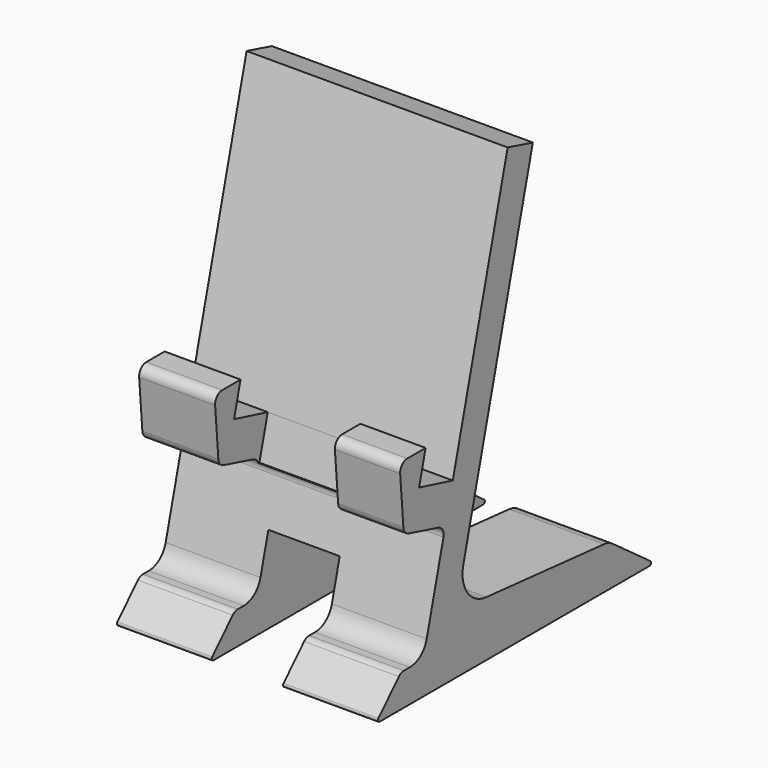
from build123d import *

# Parameters (mm, degrees)
F0_W     = 76.2
F0_H     = 101.6
F1_DEPTH = 133.35
F3_DEPTH = 76.201
F4_W     = 34.9662494294
F4_H     = 12.1309220302
F5_DEPTH = 25.4
F6_W     = 20.8403859288
F6_H     = 113.2664903998
F7_DEPTH = 25.4


# Not quite as in the source:
# - a feature names something its author has since deleted; it is built from what else it names


with BuildPart() as f1:
    # F0 (on Top) → F1 (new body)
    with BuildSketch(Plane.XY):
        Rectangle(F0_W, F0_H)
    extrude(amount=F1_DEPTH)

    # F2 (on face) → F3 (cut, through all)
    with BuildSketch(Plane.YZ.offset(38.1)):
        with BuildLine():
            Line((49.114014449, 0), (50.8, 0))
            Line((50.8, 0), (50.8, 66.2650913))
            Line((50.8, 66.2650913), (50.8, 73.7310647964))
            Line((50.8, 73.7310647964), (50.8, 128.6014442141))
            Line((50.8, 128.6014442141), (50.8, 133.35))
            Line((50.8, 133.35), (-50.8, 133.35))
            Line((-50.8, 133.35), (-50.8, 0))
            Line((-50.8, 0), (-49.3153884285, 0))
            ThreePointArc((-49.3153884285, 0), (-49.8930613229, 0.38308634), (-49.7649416709, 1.0642959051))
            Line((-49.7649416709, 1.0642959051), (-42.2846688887, 8.7558660005))
            ThreePointArc((-42.2846688887, 8.7558660005), (-41.4521127702, 9.3248290153), (-40.4637807514, 9.525))
            Line((-40.4637807514, 9.525), (-38.2985454719, 9.525))
            ThreePointArc((-38.2985454719, 9.525), (-34.4105014329, 10.8544807489), (-32.1505139925, 14.2862240786))
            Line((-32.1505139925, 14.2862240786), (-26.0325690106, 37.9606251271))
            ThreePointArc((-26.0325690106, 37.9606251271), (-26.3063034957, 39.9399780989), (-27.8936985581, 41.1536278306))
            Line((-27.8936985581, 41.1536278306), (-38.7149990474, 44.0606170611))
            ThreePointArc((-38.7149990474, 44.0606170611), (-40.050293777, 44.9146793042), (-40.6508289049, 46.3815780362))
            Line((-40.6508289049, 46.3815780362), (-41.828178264, 60.7104246977))
            ThreePointArc((-41.828178264, 60.7104246977), (-41.1424179273, 62.7046091009), (-39.2110885015, 63.5513707689))
            Line((-39.2110885015, 63.5513707689), (-32.5366084985, 63.5513707689))
            Line((-32.5366084985, 63.5513707689), (-34.9197723805, 54.3293235498))
            Line((-34.9197723805, 54.3293235498), (-22.6237094217, 51.1517717071))
            Line((-22.6237094217, 51.1517717071), (-2.6091445634, 128.6014442141))
            Line((-2.6091445634, 128.6014442141), (6.5897179326, 126.1302999894))
            Line((6.5897179326, 126.1302999894), (-18.753958765, 28.0587468857))
            ThreePointArc((-18.753958765, 28.0587468857), (-17.3156963729, 20.1857452314), (-10.3820422123, 16.1885970308))
            Line((-10.3820422123, 16.1885970308), (32.5785662344, 12.338888515))
            ThreePointArc((32.5785662344, 12.338888515), (34.2472884437, 11.9577274025), (35.7535762689, 11.144699363))
            Line((35.7535762689, 11.144699363), (49.5238091926, 1.1017641769))
            ThreePointArc((49.5238091926, 1.1017641769), (49.7017678057, 0.4084810434), (49.114014449, 0))
        make_face()
    extrude(amount=-F3_DEPTH, mode=Mode.SUBTRACT)

    # F4 (on face) → F5 (cut)
    with BuildSketch(Plane(origin=(0, -33.598613666, 8.682562632), x_dir=(1, 0, 0), z_dir=(0, -0.9681939338, 0.2502009325))):
        Polygon((19.05, 73.9268932369), (-15.9162494294, 83.0707615279), (-15.9162494294, 43.8643618742), (19.05, 43.8643618742), align=None)
        with Locations((1.5668752853, 37.7989008591)):
            Rectangle(F4_W, F4_H)
    extrude(amount=F5_DEPTH, mode=Mode.SUBTRACT)

    # F6 (on face) → F7 (cut)
    with BuildSketch(Plane(origin=(0, 0, 0), x_dir=(1, 0, 0), z_dir=(0, 0, -1))):
        Rectangle(F6_W, F6_H)
    extrude(amount=-F7_DEPTH, mode=Mode.SUBTRACT)


solid = f1.part
